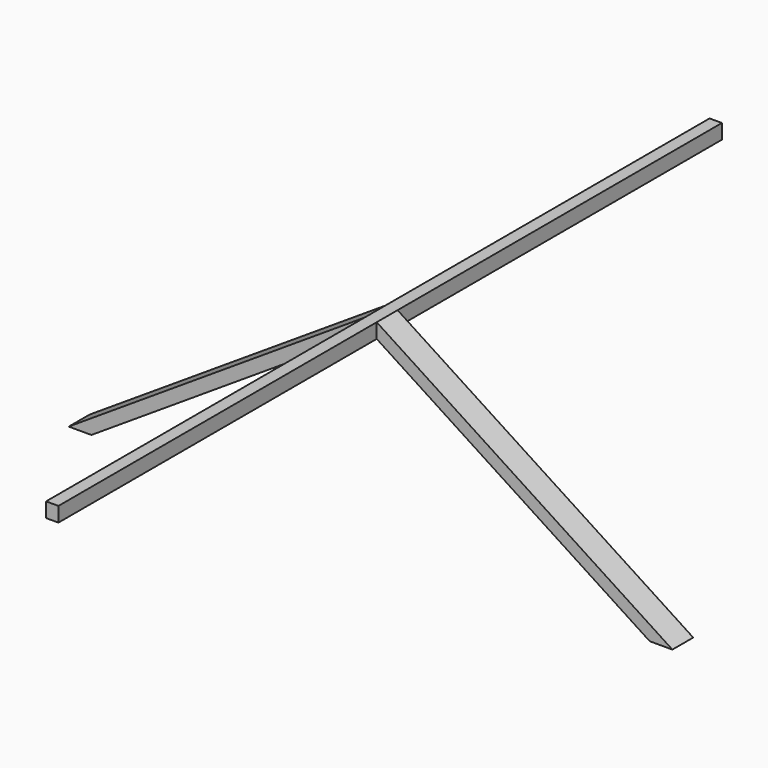
from build123d import *

# Parameters (mm, degrees)
F1_DEPTH = 95
F0_W     = 45
F0_H     = 53.6623383946
F2_DEPTH = 1477.5
F3_DEPTH = 1545


with BuildPart() as f1:
    # F0 (on Front) → F1 (new body)
    with BuildSketch(Plane.XZ):
        Polygon((-22.5, 237.5461500682), (-22.5, 291.2084884628), (-1100, -408.7915115372), (-1017.398329114, -408.7915115372), align=None)
    extrude(amount=F1_DEPTH)


with BuildPart() as f1b:
    # F0 (on Front) → F1, piece 2 (new body)
    with BuildSketch(Plane.XZ):
        Polygon((1100, -408.7915115372), (22.5, 291.2084884628), (22.5, 237.5461500682), (1017.398329114, -408.7915115372), align=None)
    extrude(amount=F1_DEPTH)


with BuildPart() as f2:
    # F0 (on Front) → F2 (new body)
    with BuildSketch(Plane.XZ):
        with Locations((0, 264.3773192655)):
            Rectangle(F0_W, F0_H)
    extrude(amount=-F2_DEPTH)

    # F0 (on Front) → F3 (join)
    with BuildSketch(Plane.XZ):
        with Locations((0, 264.3773192655)):
            Rectangle(F0_W, F0_H)
    extrude(amount=F3_DEPTH)


solid = Compound([f1.part, f1b.part, f2.part])
